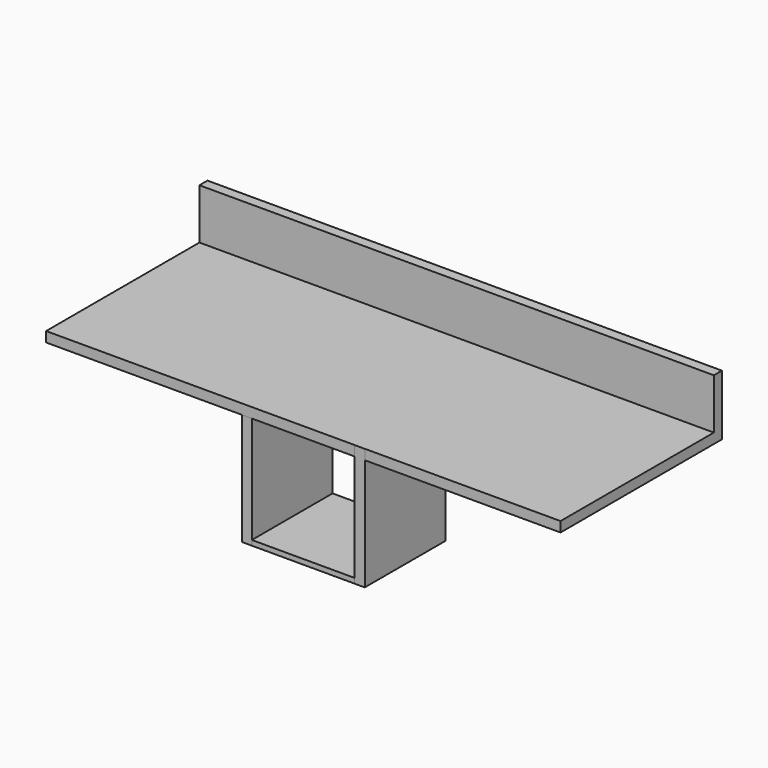
from build123d import *

# Parameters (mm, degrees)
F8_DEPTH  = 1.27
F9_DEPTH  = 2.54
F10_DEPTH = 2.54
F11_DEPTH = 2.54
F13_DEPTH = 2.54


# Not quite as in the source:
# - a feature names something its author has since deleted; it is built from what else it names


with BuildPart() as f8:
    # F3 (on offset) → F8 (new body)
    with BuildSketch(Plane.XY.offset(-28.194)):
        Polygon((0, -12.7), (0, 0), (0, 12.7), (-12.954, 12.7), (-12.954, -12.7), align=None)
        Polygon((0, 12.7), (0, 0), (0, -12.7), (12.954, -12.7), (12.954, 12.7), align=None)
    extrude(amount=F8_DEPTH)


with BuildPart() as f9:
    # F7 (on offset) → F9 (new body)
    with BuildSketch(Plane.YZ.offset(-15.494)):
        Polygon((12.7, 2.54), (0, 2.54), (-12.7, 2.54), (-12.7, -28.194), (12.7, -28.194), align=None)
    extrude(amount=F9_DEPTH)


with BuildPart() as f10:
    # F5 (on offset) → F10 (new body)
    with BuildSketch(Plane.YZ.offset(15.494)):
        Polygon((12.6734433368, 2.54), (-12.7265510293, 2.54), (-12.7265510293, -28.1820375444), (12.6734433368, -28.194), align=None)
    extrude(amount=-F10_DEPTH)


with BuildPart() as f11:
    # F0 (on Top) → F11 (new body)
    with BuildSketch(Plane.XY):
        Polygon((-64.77, 38.1), (-64.77, 0), (-64.77, -12.7), (64.77, -12.7), (64.77, 38.1), align=None)
    extrude(amount=F11_DEPTH)

    # F12 (on offset) → F13 (join)
    with BuildSketch(Plane.XZ.offset(-38.1)):
        Polygon((-64.77, 0), (0, 0), (64.77, 0), (64.77, 15.24), (-64.77, 15.24), align=None)
    extrude(amount=F13_DEPTH)


solid = Compound([f8.part, f9.part, f10.part, f11.part])
